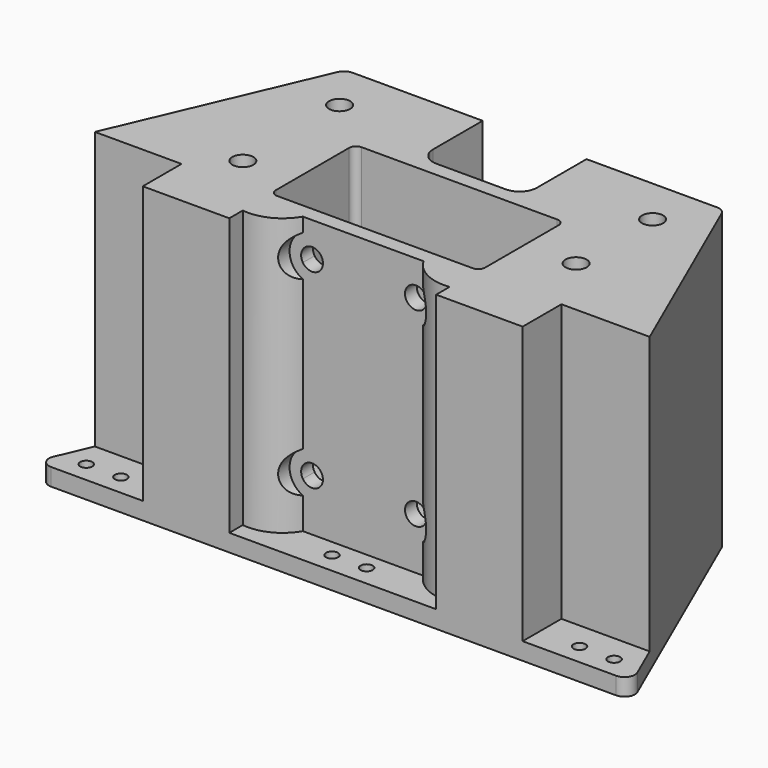
from build123d import *

# Parameters (mm, degrees)
F0_R      = 1.75
F1_DEPTH  = 5
F3_DEPTH  = 80
F2_R      = 4.15
F4_DEPTH  = 5.001
F6_DEPTH  = 25
F7_DEPTH  = 11.001
F8_R      = 5
F9_DEPTH  = 5
F10_R     = 10
F10_R_2   = 4.15
F11_DEPTH = 5.7
F12_DEPTH = 5
F15_DEPTH = 80
F13_R     = 3.05
F16_DEPTH = 85.001


# Not quite as in the source:
# - a pattern or mirror of a feature is missing from the dataset's text; its kind, count and spacing are read off the source's solid


with BuildPart() as f1:
    # F0 (on Top) → F1 (new body)
    with BuildSketch(Plane.XY):
        with BuildLine():
            ThreePointArc((-52.6663762242, 17.9), (-54.3173783407, 17.4048337293), (-55.4233667499, 16.0827946742))
            Line((-55.4233667499, 16.0827946742), (-84.1245766253, -50.8172053258))
            ThreePointArc((-84.1245766253, -50.8172053258), (-83.8724198289, -53.6510021165), (-81.3675860996, -55))
            Line((-81.3675860996, -55), (81.9025433219, -55))
            ThreePointArc((81.9025433219, -55), (84.4127764383, -53.6427810874), (84.651718981, -50.7991531341))
            Line((84.651718981, -50.7991531341), (55.429630147, 16.1008468659))
            ThreePointArc((55.429630147, 16.1008468659), (54.3232355753, 17.4102331165), (52.6804544879, 17.9))
            Line((52.6804544879, 17.9), (-52.6663762242, 17.9))
        make_face()
        with Locations((-76, -49)):
            Circle(F0_R, mode=Mode.SUBTRACT)
        with Locations((-66, -49)):
            Circle(F0_R, mode=Mode.SUBTRACT)
        with Locations((-5, -49)):
            Circle(F0_R, mode=Mode.SUBTRACT)
        with Locations((5, -49)):
            Circle(F0_R, mode=Mode.SUBTRACT)
        with Locations((66.5, -49)):
            Circle(F0_R, mode=Mode.SUBTRACT)
        with Locations((76.5, -49)):
            Circle(F0_R, mode=Mode.SUBTRACT)
        with BuildLine():
            ThreePointArc((-47.475, 1.75), (-53.625, 7.9), (-47.475, 14.05))
            Line((-47.475, 14.05), (-23.025, 14.05))
            ThreePointArc((-23.025, 14.05), (-16.875, 7.9), (-23.025, 1.75))
            Line((-23.025, 1.75), (-47.475, 1.75))
        make_face(mode=Mode.SUBTRACT)
        with Locations((-5, 0)):
            Circle(F0_R, mode=Mode.SUBTRACT)
        with Locations((5, 0)):
            Circle(F0_R, mode=Mode.SUBTRACT)
        with BuildLine():
            ThreePointArc((23.15, 1.75), (17, 7.9), (23.15, 14.05))
            Line((23.15, 14.05), (47.35, 14.05))
            ThreePointArc((47.35, 14.05), (53.5, 7.9), (47.35, 1.75))
            Line((47.35, 1.75), (23.15, 1.75))
        make_face(mode=Mode.SUBTRACT)
        with BuildLine():
            Line((-23.025, 14.05), (-47.475, 14.05))
            ThreePointArc((-47.475, 14.05), (-53.625, 7.9), (-47.475, 1.75))
            Line((-47.475, 1.75), (-23.025, 1.75))
            ThreePointArc((-23.025, 1.75), (-16.875, 7.9), (-23.025, 14.05))
        make_face()
        with BuildLine():
            Line((47.35, 14.05), (23.15, 14.05))
            ThreePointArc((23.15, 14.05), (17, 7.9), (23.15, 1.75))
            Line((23.15, 1.75), (47.35, 1.75))
            ThreePointArc((47.35, 1.75), (53.5, 7.9), (47.35, 14.05))
        make_face()
    extrude(amount=F1_DEPTH)

    # F2 (on face) → F3 (join)
    with BuildSketch(Plane.XY.offset(5)):
        with BuildLine():
            ThreePointArc((-52.6663762242, 17.9), (-54.3173783407, 17.4048337293), (-55.4233667499, 16.0827946742))
            Line((-55.4233667499, 16.0827946742), (-79.9128326725, -41))
            Line((-79.9128326725, -41), (-40.3201077046, -41))
            ThreePointArc((-40.3201077046, -41), (-29.8739998873, -50.1440560095), (-17.4246824527, -44))
            Line((-17.4246824527, -44), (17.4246824527, -44))
            ThreePointArc((17.4246824527, -44), (29.8739998873, -50.1440560095), (40.3201077046, -41))
            Line((40.3201077046, -41), (80.3714241621, -41))
            Line((80.3714241621, -41), (55.429630147, 16.1008468659))
            ThreePointArc((55.429630147, 16.1008468659), (54.3232355753, 17.4102331165), (52.6804544879, 17.9))
            Line((52.6804544879, 17.9), (15, 17.9))
            Line((15, 17.9), (15, -5))
            Line((15, -5), (-15, -5))
            Line((-15, -5), (-15, 17.9))
            Line((-15, 17.9), (-52.6663762242, 17.9))
        make_face()
        with BuildLine():
            ThreePointArc((-30.25, -11.25), (-29.6642135624, -9.8357864376), (-28.25, -9.25))
            Line((-28.25, -9.25), (28.25, -9.25))
            ThreePointArc((28.25, -9.25), (29.6642135624, -9.8357864376), (30.25, -11.25))
            Line((30.25, -11.25), (30.25, -37.75))
            ThreePointArc((30.25, -37.75), (29.6642135624, -39.1642135624), (28.25, -39.75))
            Line((28.25, -39.75), (-28.25, -39.75))
            ThreePointArc((-28.25, -39.75), (-29.6642135624, -39.1642135624), (-30.25, -37.75))
            Line((-30.25, -37.75), (-30.25, -11.25))
        make_face(mode=Mode.SUBTRACT)
    extrude(amount=F3_DEPTH)

    # F2 (on face) → F4 (cut, through all)
    with BuildSketch(Plane.XY.offset(5)):
        with Locations((-15, -24.5)):
            Circle(F2_R)
        with Locations((15, -24.5)):
            Circle(F2_R)
    extrude(amount=-F4_DEPTH, mode=Mode.SUBTRACT)

    # F5 (on face) → F6 (cut)
    with BuildSketch(Plane.XZ.offset(44)):
        with BuildLine():
            ThreePointArc((-17.4246824527, 73.3032679271), (-13.886829638, 71.9765473939), (-11.6207042552, 75))
            ThreePointArc((-11.6207042552, 75), (-13.886829638, 78.0234526061), (-17.4246824527, 76.6967320729))
            Line((-17.4246824527, 76.6967320729), (-17.4246824527, 73.3032679271))
        make_face()
        with BuildLine():
            ThreePointArc((18.3792957448, 75), (18.1308443081, 76.2261794058), (17.4246824527, 77.2589327575))
            Line((17.4246824527, 77.2589327575), (17.4246824527, 72.7410672425))
            ThreePointArc((17.4246824527, 72.7410672425), (18.1308443081, 73.7738205942), (18.3792957448, 75))
        make_face()
        with BuildLine():
            Line((17.4246824527, 17.7410672425), (17.4246824527, 22.2589327575))
            ThreePointArc((17.4246824527, 22.2589327575), (12.0792957448, 20), (17.4246824527, 17.7410672425))
        make_face()
        with BuildLine():
            Line((-17.4246824527, 18.3032679271), (-17.4246824527, 21.6967320729))
            ThreePointArc((-17.4246824527, 21.6967320729), (-17.9207042552, 20), (-17.4246824527, 18.3032679271))
        make_face()
        with BuildLine():
            ThreePointArc((-11.6207042552, 20), (-13.886829638, 23.0234526061), (-17.4246824527, 21.6967320729))
            Line((-17.4246824527, 21.6967320729), (-17.4246824527, 18.3032679271))
            ThreePointArc((-17.4246824527, 18.3032679271), (-13.886829638, 16.9765473939), (-11.6207042552, 20))
        make_face()
        with BuildLine():
            Line((-17.4246824527, 73.3032679271), (-17.4246824527, 76.6967320729))
            ThreePointArc((-17.4246824527, 76.6967320729), (-17.9207042552, 75), (-17.4246824527, 73.3032679271))
        make_face()
        with BuildLine():
            Line((17.4246824527, 72.7410672425), (17.4246824527, 77.2589327575))
            ThreePointArc((17.4246824527, 77.2589327575), (12.0792957448, 75), (17.4246824527, 72.7410672425))
        make_face()
        with BuildLine():
            ThreePointArc((18.3792957448, 20), (18.1308443081, 21.2261794058), (17.4246824527, 22.2589327575))
            Line((17.4246824527, 22.2589327575), (17.4246824527, 17.7410672425))
            ThreePointArc((17.4246824527, 17.7410672425), (18.1308443081, 18.7738205942), (18.3792957448, 20))
        make_face()
    extrude(amount=-F6_DEPTH, mode=Mode.SUBTRACT)

    # F5 (on face) → F7 (cut, through all)
    with BuildSketch(Plane.XZ.offset(44)):
        with BuildLine():
            Line((17.4246824527, 72.7410672425), (17.4246824527, 77.2589327575))
            ThreePointArc((17.4246824527, 77.2589327575), (12.0792957448, 75), (17.4246824527, 72.7410672425))
        make_face()
        with BuildLine():
            Line((17.4246824527, 77.2589327575), (17.4246824527, 81.1180288658))
            ThreePointArc((17.4246824527, 81.1180288658), (8.7292957448, 75), (17.4246824527, 68.8819711342))
            Line((17.4246824527, 68.8819711342), (17.4246824527, 72.7410672425))
            ThreePointArc((17.4246824527, 72.7410672425), (12.0792957448, 75), (17.4246824527, 77.2589327575))
        make_face()
        with BuildLine():
            ThreePointArc((21.7292957448, 20), (20.5453099285, 23.7403199328), (17.4246824527, 26.1180288658))
            Line((17.4246824527, 26.1180288658), (17.4246824527, 22.2589327575))
            ThreePointArc((17.4246824527, 22.2589327575), (18.1308443081, 21.2261794058), (18.3792957448, 20))
            ThreePointArc((18.3792957448, 20), (18.1308443081, 18.7738205942), (17.4246824527, 17.7410672425))
            Line((17.4246824527, 17.7410672425), (17.4246824527, 13.8819711342))
            ThreePointArc((17.4246824527, 13.8819711342), (20.5453099285, 16.2596800672), (21.7292957448, 20))
        make_face()
        with BuildLine():
            Line((-17.4246824527, 73.3032679271), (-17.4246824527, 76.6967320729))
            ThreePointArc((-17.4246824527, 76.6967320729), (-17.9207042552, 75), (-17.4246824527, 73.3032679271))
        make_face()
        with BuildLine():
            ThreePointArc((-11.6207042552, 20), (-13.886829638, 23.0234526061), (-17.4246824527, 21.6967320729))
            Line((-17.4246824527, 21.6967320729), (-17.4246824527, 18.3032679271))
            ThreePointArc((-17.4246824527, 18.3032679271), (-13.886829638, 16.9765473939), (-11.6207042552, 20))
        make_face()
        with BuildLine():
            ThreePointArc((18.3792957448, 20), (18.1308443081, 21.2261794058), (17.4246824527, 22.2589327575))
            Line((17.4246824527, 22.2589327575), (17.4246824527, 17.7410672425))
            ThreePointArc((17.4246824527, 17.7410672425), (18.1308443081, 18.7738205942), (18.3792957448, 20))
        make_face()
        with BuildLine():
            ThreePointArc((-8.2707042552, 20), (-11.2352310396, 25.4543953966), (-17.4246824527, 25.9334981021))
            Line((-17.4246824527, 25.9334981021), (-17.4246824527, 21.6967320729))
            ThreePointArc((-17.4246824527, 21.6967320729), (-13.886829638, 23.0234526061), (-11.6207042552, 20))
            ThreePointArc((-11.6207042552, 20), (-13.886829638, 16.9765473939), (-17.4246824527, 18.3032679271))
            Line((-17.4246824527, 18.3032679271), (-17.4246824527, 14.0665018979))
            ThreePointArc((-17.4246824527, 14.0665018979), (-11.2352310396, 14.5456046034), (-8.2707042552, 20))
        make_face()
        with BuildLine():
            ThreePointArc((-17.4246824527, 73.3032679271), (-17.9207042552, 75), (-17.4246824527, 76.6967320729))
            Line((-17.4246824527, 76.6967320729), (-17.4246824527, 80.9334981021))
            ThreePointArc((-17.4246824527, 80.9334981021), (-21.2707042552, 75), (-17.4246824527, 69.0665018979))
            Line((-17.4246824527, 69.0665018979), (-17.4246824527, 73.3032679271))
        make_face()
    f7 = extrude(amount=F7_DEPTH, mode=Mode.SUBTRACT)

    # F7_copies: F7 across plane
    add(f7.mirror(Plane(origin=(-1.2e-05, 2.3e-05, 47.499983), x_dir=(1, 0, 0), z_dir=(0, 0, 1))), mode=Mode.SUBTRACT)

    # F8
    f8_edges = [f1.edges().sort_by_distance(p)[0] for p in [
        (-15, -5, 45),
        (15, -5, 45),
    ]]
    fillet(f8_edges, radius=F8_R)

    # F2 (on face) → F9 (join)
    with BuildSketch(Plane.XY.offset(5)):
        with BuildLine():
            Line((28.25, -9.25), (-28.25, -9.25))
            ThreePointArc((-28.25, -9.25), (-29.6642135624, -9.8357864376), (-30.25, -11.25))
            Line((-30.25, -11.25), (-30.25, -37.75))
            ThreePointArc((-30.25, -37.75), (-29.6642135624, -39.1642135624), (-28.25, -39.75))
            Line((-28.25, -39.75), (28.25, -39.75))
            ThreePointArc((28.25, -39.75), (29.6642135624, -39.1642135624), (30.25, -37.75))
            Line((30.25, -37.75), (30.25, -11.25))
            ThreePointArc((30.25, -11.25), (29.6642135624, -9.8357864376), (28.25, -9.25))
        make_face()
        with Locations((-15, -24.5)):
            Circle(F2_R, mode=Mode.SUBTRACT)
        with Locations((15, -24.5)):
            Circle(F2_R, mode=Mode.SUBTRACT)
    extrude(amount=F9_DEPTH)

    # F10 (on face) → F11 (cut)
    with BuildSketch(Plane(origin=(0, 0, 0), x_dir=(1, 0, 0), z_dir=(0, 0, -1))):
        with Locations((-15, 24.5)):
            Circle(F10_R)
        with Locations((-15, 24.5)):
            Circle(F10_R_2, mode=Mode.SUBTRACT)
        with Locations((15, 24.5)):
            Circle(F10_R)
        with Locations((15, 24.5)):
            Circle(F10_R_2, mode=Mode.SUBTRACT)
    extrude(amount=-F11_DEPTH, mode=Mode.SUBTRACT)

    # F0 (on Top) → F12 (cut)
    with BuildSketch(Plane.XY):
        with BuildLine():
            Line((-23.025, 14.05), (-47.475, 14.05))
            ThreePointArc((-47.475, 14.05), (-53.625, 7.9), (-47.475, 1.75))
            Line((-47.475, 1.75), (-23.025, 1.75))
            ThreePointArc((-23.025, 1.75), (-16.875, 7.9), (-23.025, 14.05))
        make_face()
        with BuildLine():
            Line((47.35, 14.05), (23.15, 14.05))
            ThreePointArc((23.15, 14.05), (17, 7.9), (23.15, 1.75))
            Line((23.15, 1.75), (47.35, 1.75))
            ThreePointArc((47.35, 1.75), (53.5, 7.9), (47.35, 14.05))
        make_face()
    extrude(amount=F12_DEPTH, mode=Mode.SUBTRACT)

    # F14 (on face) → F15 (join, through all)
    with BuildSketch(Plane.XY.offset(5)):
        with BuildLine():
            Line((-40.3201077046, -41), (-54.8739998873, -41))
            Line((-54.8739998873, -41), (-54.8739998873, -55))
            Line((-54.8739998873, -55), (-29.8739998873, -55))
            Line((-29.8739998873, -55), (-29.8739998873, -50.1440560095))
            ThreePointArc((-29.8739998873, -50.1440560095), (-36.4832002138, -47.1555523091), (-40.3201077046, -41))
        make_face()
        with BuildLine():
            Line((29.8739998873, -50.1440560095), (29.8739998873, -55))
            Line((29.8739998873, -55), (54.8739998873, -55))
            Line((54.8739998873, -55), (54.8739998873, -41))
            Line((54.8739998873, -41), (40.3201077046, -41))
            ThreePointArc((40.3201077046, -41), (36.4832002138, -47.1555523091), (29.8739998873, -50.1440560095))
        make_face()
    extrude(amount=F15_DEPTH)

    # F13 (on face) → F16 (cut, through all)
    with BuildSketch(Plane.XY.offset(85)):
        with Locations((-45, 3.7425805349)):
            Circle(F13_R)
        with Locations((-45, -31.2046017498)):
            Circle(F13_R)
        with Locations((45, 4.2540011927)):
            Circle(F13_R)
        with Locations((45, -23.362794891)):
            Circle(F13_R)
    extrude(amount=-F16_DEPTH, mode=Mode.SUBTRACT)


solid = f1.part
